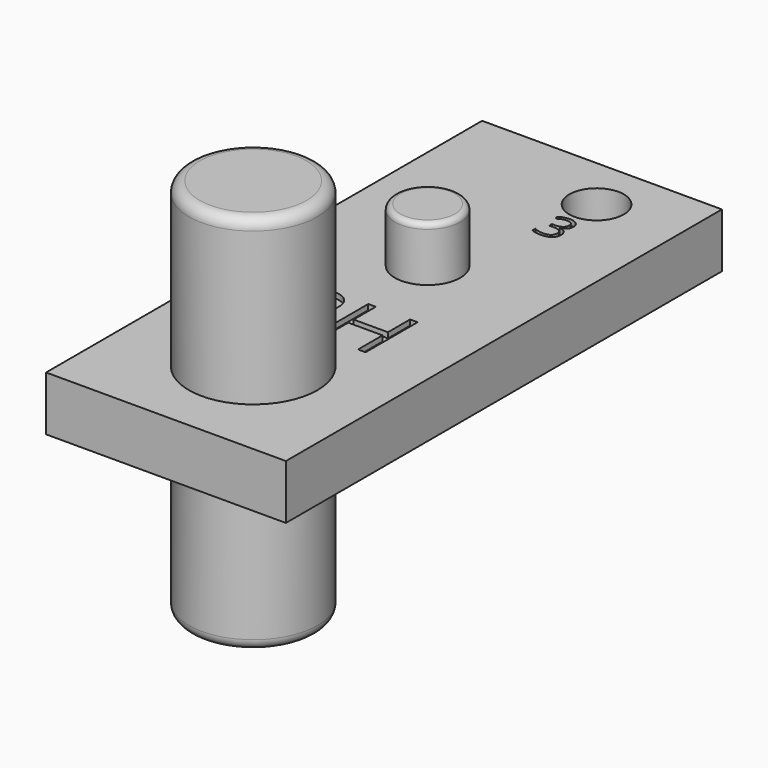
from build123d import *

# Parameters (mm, degrees)
F0_W          = 22
F0_H          = 50
F1_DEPTH      = 5
F2_R          = 5.9
F3_DEPTH      = 15
F3_DEPTH_BACK = 20
F4_R          = 3
F5_DEPTH      = 5
F5_DEPTH_BACK = 10
F6_R          = 2.5
F7_DEPTH      = 20.001
F9_TEXT_SIZE  = 8.3557407682
F10_DEPTH     = 0.5
F8_TEXT_SIZE  = 4.3821950062
F11_DEPTH     = 0.5
F12_TEXT_SIZE = 10.0457880439
F13_DEPTH     = 0.5
F14_TEXT_SIZE = 3.8923488723
F15_DEPTH     = 0.5
F16_R         = 1
F17_R         = 0.5


# Not quite as in the source:
# - Text() gives the source's letters only with a copy of the font that has no kerning and outlines rounded to 1/6400 em; it was checked with that copy


with BuildPart() as f1:
    # F0 (on Top) → F1 (new body)
    with BuildSketch(Plane.XY):
        with Locations((11, 25)):
            Rectangle(F0_W, F0_H)
    extrude(amount=F1_DEPTH)

    # F2 (on face) → F3 (join, two sides)
    with BuildSketch(Plane.XY.offset(5)) as f3_sk:
        with Locations((11, 10)):
            Circle(F2_R)
    extrude(amount=F3_DEPTH)
    extrude(f3_sk.sketch, amount=-F3_DEPTH_BACK)

    # F4 (on face) → F5 (join, two sides)
    with BuildSketch(Plane.XY.offset(5)) as f5_sk:
        with Locations((11, 30)):
            Circle(F4_R)
    extrude(amount=F5_DEPTH)
    extrude(f5_sk.sketch, amount=-F5_DEPTH_BACK)

    # F6 (on face) → F7 (cut, through all)
    with BuildSketch(Plane.XY.offset(5)):
        with Locations((14.5, 45)):
            Circle(F6_R)
    extrude(amount=-F7_DEPTH, mode=Mode.SUBTRACT)

    # F9 (on face) → F10 (cut)
    with BuildSketch(Plane.XY.offset(5)):
        with Locations((5.4005142301, 16.7460031807)):
            Text('RH', F9_TEXT_SIZE, font='Open Sans', text_align=(TextAlign.LEFT, TextAlign.BOTTOM))
    extrude(amount=-F10_DEPTH, mode=Mode.SUBTRACT)

    # F8 (on face) → F11 (cut)
    with BuildSketch(Plane.XY.offset(5)):
        with Locations((13.233614115, 38.8448195956)):
            Text('3', F8_TEXT_SIZE, font='Open Sans', text_align=(TextAlign.LEFT, TextAlign.BOTTOM))
    extrude(amount=-F11_DEPTH, mode=Mode.SUBTRACT)

    # F12 (on face) → F13 (cut)
    with BuildSketch(Plane(origin=(0, 0, 0), x_dir=(1, 0, 0), z_dir=(0, 0, -1))):
        with Locations((4.5243469067, -25)):
            Text('LH', F12_TEXT_SIZE, font='Open Sans', text_align=(TextAlign.LEFT, TextAlign.BOTTOM))
    extrude(amount=-F13_DEPTH, mode=Mode.SUBTRACT)

    # F14 (on face) → F15 (cut)
    with BuildSketch(Plane(origin=(0, 0, 0), x_dir=(1, 0, 0), z_dir=(0, 0, -1))):
        with Locations((13.3751719939, -41.1966219544)):
            Text('3', F14_TEXT_SIZE, font='Open Sans', text_align=(TextAlign.LEFT, TextAlign.BOTTOM))
    extrude(amount=-F15_DEPTH, mode=Mode.SUBTRACT)

    # F16
    f16_edges = [f1.edges().sort_by_distance(p)[0] for p in [
        (5.1, 10, 20),
        (5.1, 10, -15),
    ]]
    fillet(f16_edges, radius=F16_R)

    # F17
    f17_edges = [f1.edges().sort_by_distance(p)[0] for p in [
        (8, 30, 10),
        (8, 30, -5),
    ]]
    fillet(f17_edges, radius=F17_R)


solid = f1.part
